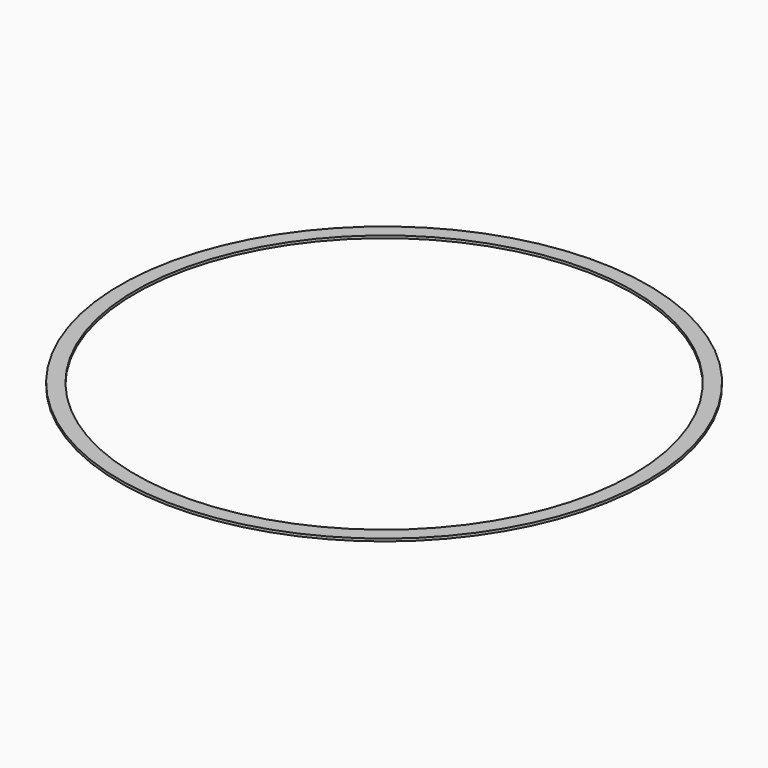
from build123d import *

# Parameters (mm, degrees)
F0_R     = 444.50127
F0_R_2   = 419.10127
F1_DEPTH = 4.2333333333


# Not quite as in the source:
# - a length typed as a fraction of an inch, garbled in the dataset ("3 / 203.2 mm" for 3/8 in), is restored


with BuildPart() as f1:
    # F0 (on Top) → F1 (new body)
    with BuildSketch(Plane.XY):
        Circle(F0_R)
        Circle(F0_R_2, mode=Mode.SUBTRACT)
    extrude(amount=F1_DEPTH)


solid = f1.part
